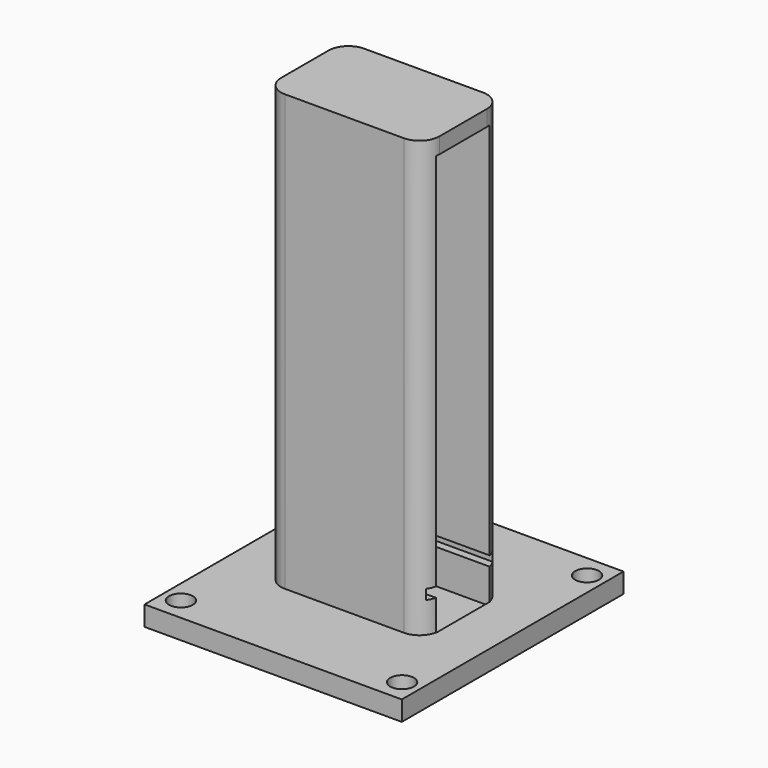
from build123d import *

# Parameters (mm, degrees)
F0_W         = 65
F0_H         = 70
F1_DEPTH     = 5
F2_W         = 40
F2_H         = 25
F3_DEPTH     = 110
F5_D         = 6
F6_T         = -4
F7_W         = 7.9657556489
F7_H         = 25
F8_DEPTH     = 25
F10_DEPTH    = 2
F11_T1_DEPTH = 122.5


# Not quite as in the source:
# - a fillet or chamfer that OpenCascade refuses, or shapes differently, is made with other operations: its cross-section is extruded or revolved along the edge and cut away or added
# - a pattern or mirror of a feature is missing from the dataset's text; its kind, count and spacing are read off the source's solid


with BuildPart() as f1:
    # F0 (on Top) → F1 (new body)
    with BuildSketch(Plane.XY):
        Rectangle(F0_W, F0_H)
    extrude(amount=F1_DEPTH)

    # F2 (on face) → F3 (join)
    with BuildSketch(Plane.XY.offset(5)):
        Rectangle(F2_W, F2_H)
    extrude(amount=F3_DEPTH)

    # F5 (through all)
    with Locations(Plane(origin=(0, 0, 0), x_dir=(1, 0, 0), z_dir=(0, 0, -1))):
        with Locations((-27.94, 29.21), (27.94, 29.21), (27.94, -29.21), (-27.94, -29.21)):
            Hole(F5_D / 2)

    # F6: a shell. OpenCascade refuses it in one call, so the cavity is built on its own and cut out:
    # the body offset inwards by the wall thickness, plus a prism from it out through each open face.
    f6_core = offset(f1.part, amount=F6_T, kind=Kind.INTERSECTION, mode=Mode.PRIVATE)
    f6_exits = [f6_core.faces().sort_by_distance(p)[0] for p in [
        (16, 0, 57.5),
    ]]
    add(f6_core, mode=Mode.SUBTRACT)
    extrude(f6_exits, amount=-F6_T, mode=Mode.SUBTRACT)

    # F7 (on face) → F8 (cut)
    with BuildSketch(Plane.YZ.offset(-16)):
        with Locations((0, 24)):
            Rectangle(F7_W, F7_H)
    extrude(amount=-F8_DEPTH, mode=Mode.SUBTRACT)

    # F9 (on face) → F10 (cut)
    with BuildSketch(Plane.XZ.offset(-8.5)):
        with BuildLine():
            Line((20, 14), (20, 15.25))
            Line((20, 15.25), (-10, 15.25))
            ThreePointArc((-10, 15.25), (-11.25, 14), (-10, 12.75))
            Line((-10, 12.75), (20, 12.75))
            Line((20, 12.75), (20, 14))
        make_face()
    f10 = extrude(amount=-F10_DEPTH, mode=Mode.SUBTRACT)

    # F10_copies: F10 across plane
    add(f10.mirror(Plane(origin=(0, 0, 0), x_dir=(0, 0, -1), z_dir=(0, -1, 0))), mode=Mode.SUBTRACT)

    # F11: fillet of radius 5 on 4 edges, made by hand

    # F11_s2 → F11_t1 (cut)
    with BuildSketch(Plane.XY.offset(5)):
        with BuildLine():
            ThreePointArc((-15, -12.5), (-18.5355339059, -11.0355339059), (-20, -7.5))
            Line((-20, -7.5), (-20, -12.5))
            Line((-20, -12.5), (-15, -12.5))
        make_face()
        with BuildLine():
            ThreePointArc((-20, 7.5), (-18.5355339059, 11.0355339059), (-15, 12.5))
            Line((-15, 12.5), (-20, 12.5))
            Line((-20, 12.5), (-20, 7.5))
        make_face()
        with BuildLine():
            ThreePointArc((15, -12.5), (18.5355339059, -11.0355339059), (20, -7.5))
            Line((20, -7.5), (20, -12.5))
            Line((20, -12.5), (15, -12.5))
        make_face()
        with BuildLine():
            ThreePointArc((20, 7.5), (18.5355339059, 11.0355339059), (15, 12.5))
            Line((15, 12.5), (20, 12.5))
            Line((20, 12.5), (20, 7.5))
        make_face()
    extrude(amount=F11_T1_DEPTH, mode=Mode.SUBTRACT)


solid = f1.part
